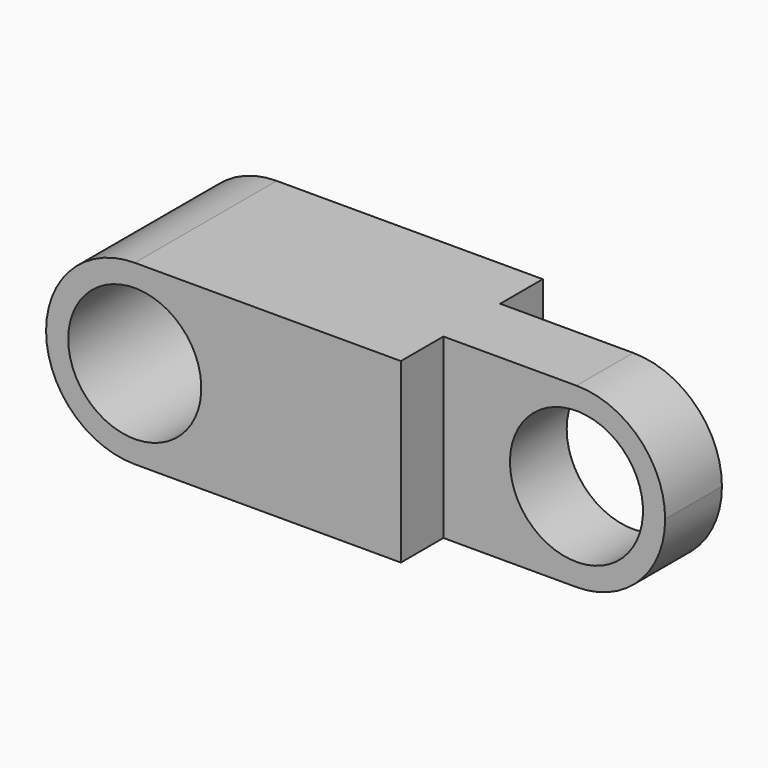
from build123d import *

# Parameters (mm, degrees)
F1_DEPTH = 5.08
F2_R     = 2.53999
F3_R     = 1.905
F4_DEPTH = 25.4
F5_R     = 1.905
F6_DEPTH = 5.08


# Not quite as in the source:
# - a fillet or chamfer is up to 0.001 mm smaller than in the source, because OpenCascade refuses the exact size


with BuildPart() as f1:
    # F0 (on Top) → F1 (new body)
    with BuildSketch(Plane.XY):
        Polygon((10.16, 0), (0, 0), (0, -5.08), (10.16, -5.08), (10.16, -3.556), (16.51, -3.556), (16.51, -1.524), (10.16, -1.524), align=None)
    extrude(amount=F1_DEPTH)

    # F2 (radius 2.54 in the source; OpenCascade refuses exactly that, so slightly less here)
    f2_edges = [f1.edges().sort_by_distance(p)[0] for p in [
        (16.51, -2.54, 5.08),
        (16.51, -2.54, 0),
        (0, -2.54, 5.08),
        (0, -2.54, 0),
    ]]
    fillet(f2_edges, radius=F2_R)

    # F3 (on face) → F4 (cut)
    with BuildSketch(Plane(origin=(0, -1.524, 0), x_dir=(-1, 0, 0), z_dir=(0, 1, 0))):
        with Locations((-13.97, 2.54)):
            Circle(F3_R)
    extrude(amount=-F4_DEPTH, mode=Mode.SUBTRACT)

    # F5 (on face) → F6 (cut)
    with BuildSketch(Plane(origin=(0, 0, 0), x_dir=(-1, 0, 0), z_dir=(0, 1, 0))):
        with Locations((-2.54, 2.54)):
            Circle(F5_R)
    extrude(amount=-F6_DEPTH, mode=Mode.SUBTRACT)


solid = f1.part
